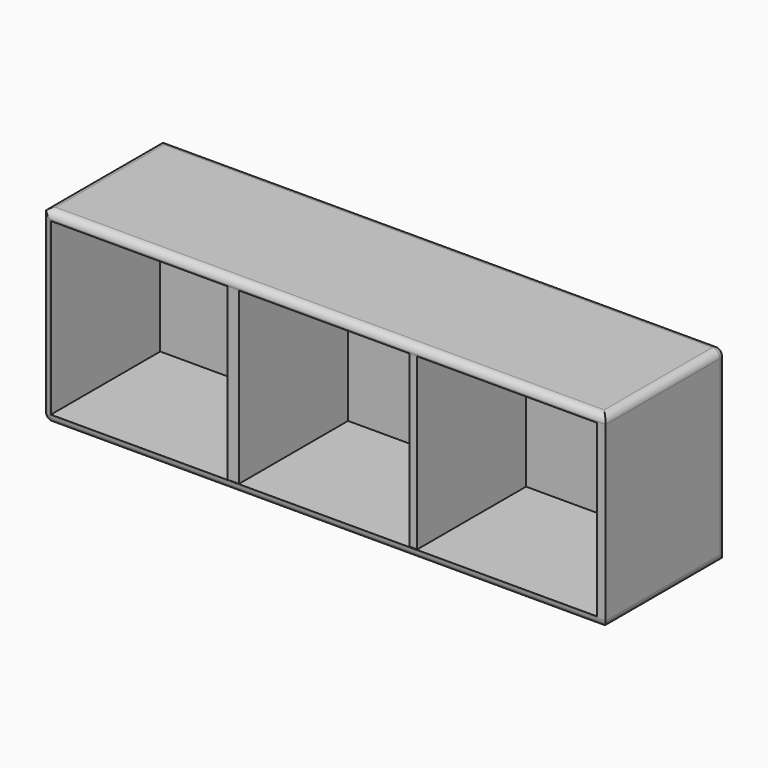
from build123d import *

# Parameters (mm, degrees)
F0_W         = 381
F0_H         = 101.6
F1_DEPTH     = 127
F2_W         = 369.2652
F2_H         = 115.2652
F3_DEPTH     = 92.456
F4_W         = 7.62
F4_H         = 115.2652
F5_DEPTH     = 92.202
F6_W         = 5.08
F6_H         = 115.2652
F7_DEPTH     = 91.948
F8_R         = 5.08
F9_T1_DEPTH  = 383.54
F9_T3_DEPTH  = 109.22
F9_T5_DEPTH  = 401.32
F9_T7_DEPTH  = 129.54
F9_S11_W     = 5.1816
F9_S11_H     = 5.1816
F9_T12_DEPTH = 5.1816


# Not quite as in the source:
# - a fillet or chamfer that OpenCascade refuses, or shapes differently, is made with other operations: its cross-section is extruded or revolved along the edge and cut away or added


with BuildPart() as f1:
    # F0 (on Top) → F1 (new body)
    with BuildSketch(Plane.XY):
        Rectangle(F0_W, F0_H)
    extrude(amount=F1_DEPTH)

    # F2 (on face) → F3 (cut)
    with BuildSketch(Plane.XZ.offset(50.8)):
        with Locations((0, 63.5)):
            Rectangle(F2_W, F2_H)
    extrude(amount=-F3_DEPTH, mode=Mode.SUBTRACT)

    # F4 (on face) → F5 (join)
    with BuildSketch(Plane.XZ.offset(-41.656)):
        with Locations((-61.4426, 63.5)):
            Rectangle(F4_W, F4_H)
    extrude(amount=F5_DEPTH)

    # F6 (on face) → F7 (join)
    with BuildSketch(Plane.XZ.offset(-41.656)):
        with Locations((60.1726, 63.5)):
            Rectangle(F6_W, F6_H)
    extrude(amount=F7_DEPTH)

    # F8
    f8_edges = [f1.edges().sort_by_distance(p)[0] for p in [
        (0, 50.8, 0),
        (-190.5, 0, 0),
        (0, -50.8, 0),
        (190.5, 0, 0),
        (-190.5, 50.8, 63.5),
        (-190.5, -50.8, 63.5),
        (-190.5, 0, 127),
    ]]
    fillet(f8_edges, radius=F8_R)

    # F9: fillet of radius 5.08 on 7 edges, made by hand

    # F9_s2 → F9_t1 (cut)
    with BuildSketch(Plane.YZ.offset(-198.12)):
        with BuildLine():
            ThreePointArc((50.8, 121.92), (49.3121024484, 125.5121024484), (45.72, 127))
            Line((45.72, 127), (50.8, 127))
            Line((50.8, 127), (50.8, 121.92))
        make_face()
    extrude(amount=F9_T1_DEPTH, mode=Mode.SUBTRACT)

    # F9_s4 → F9_t3 (cut)
    with BuildSketch(Plane.XZ.offset(-45.72)):
        with BuildLine():
            ThreePointArc((190.5, 121.92), (189.0121024484, 125.5121024484), (185.42, 127))
            Line((185.42, 127), (190.5, 127))
            Line((190.5, 127), (190.5, 121.92))
        make_face()
    extrude(amount=F9_T3_DEPTH, mode=Mode.SUBTRACT)

    # F9_s6 → F9_t5 (cut)
    with BuildSketch(Plane.YZ.offset(-198.12)):
        with BuildLine():
            ThreePointArc((-45.72, 127), (-49.3121024484, 125.5121024484), (-50.8, 121.92))
            Line((-50.8, 121.92), (-50.8, 127))
            Line((-50.8, 127), (-45.72, 127))
        make_face()
    extrude(amount=F9_T5_DEPTH, mode=Mode.SUBTRACT)

    # F9_s8 → F9_t7 (cut)
    with BuildSketch(Plane.XY.offset(-7.62)):
        with BuildLine():
            ThreePointArc((185.42, 50.8), (189.0121024484, 49.3121024484), (190.5, 45.72))
            Line((190.5, 45.72), (190.5, 50.8))
            Line((190.5, 50.8), (185.42, 50.8))
        make_face()
    extrude(amount=F9_T7_DEPTH, mode=Mode.SUBTRACT)


with BuildPart() as f9_tool10:
    # F9_s11 → F9_t12 (new body)
    with BuildSketch(Plane.XZ.offset(-45.72)):
        with Locations((188.0108, 124.5108)):
            Rectangle(F9_S11_W, F9_S11_H)
    extrude(amount=-F9_T12_DEPTH)

    # F9_s13 → F9_t14 (revolve, cut)
    with BuildSketch(Plane(origin=(185.42, 45.72, 121.92), x_dir=(-0.7071067812, 0, -0.7071067812), z_dir=(0.7071067812, 0, -0.7071067812))):
        with BuildLine():
            ThreePointArc((0, -5.08), (5.08, 0), (0, 5.08))
            Line((0, 5.08), (0, -5.08))
        make_face()
    revolve(axis=Axis((185.42, 45.72, 121.92), (0, 1, 0)), mode=Mode.SUBTRACT)


with BuildPart() as f1_1:
    add(f1.part)

    # F9_t9: cut F9_tool10
    add(f9_tool10.part, mode=Mode.SUBTRACT)


solid = f1_1.part
